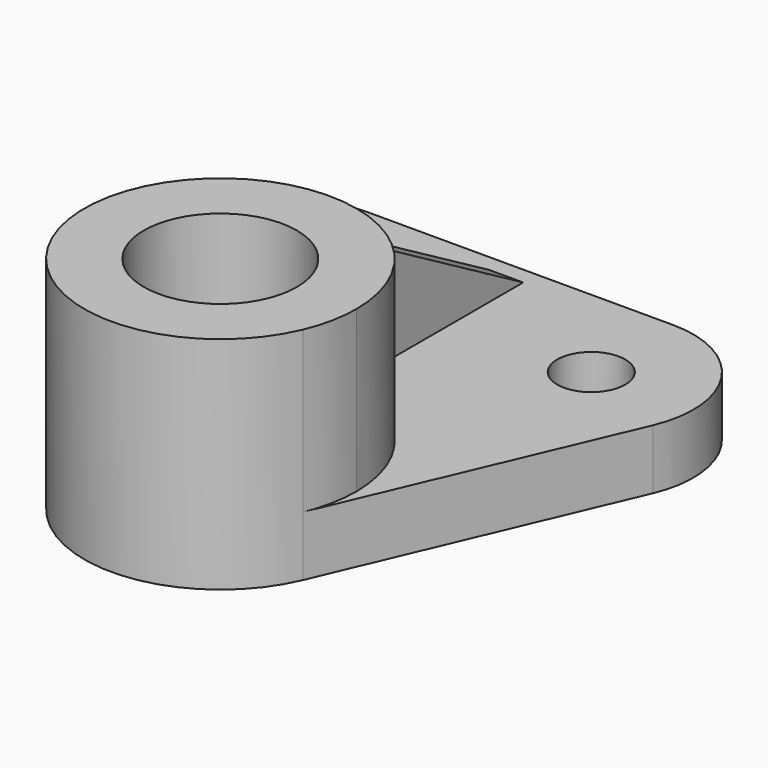
from build123d import *

# Parameters (mm, degrees)
F0_R     = 14.2875
F1_DEPTH = 41.148
F0_R_2   = 6.35
F2_DEPTH = 11.176
F4_DEPTH = 3.175


# Not quite as in the source:
# - a feature of the source that left no trace in its solid (it failed there, or was rolled back) is left out


with BuildPart() as f1:
    # F0 (on Top) → F1 (new body)
    with BuildSketch(Plane.XY):
        with BuildLine():
            ThreePointArc((23.3629201096, -9.9666425617), (24.8855195926, -5.0863458994), (25.4, 0))
            ThreePointArc((25.4, 0), (-5.0863458994, 24.8855195926), (-23.3629201096, -9.9666425617))
            ThreePointArc((-23.3629201096, -9.9666425617), (0, -25.4), (23.3629201096, -9.9666425617))
        make_face()
        Circle(F0_R, mode=Mode.SUBTRACT)
    extrude(amount=F1_DEPTH)

    # F0 (on Top) → F2 (join)
    with BuildSketch(Plane.XY):
        with BuildLine():
            ThreePointArc((-23.3629201096, -9.9666425617), (-5.0863458994, 24.8855195926), (25.4, 0))
            ThreePointArc((25.4, 0), (24.8855195926, -5.0863458994), (23.3629201096, -9.9666425617))
            Line((23.3629201096, -9.9666425617), (46.0971900822, 43.3250180788))
            ThreePointArc((46.0971900822, 43.3250180788), (44.4699820006, 61.3000974853), (28.575, 69.85))
            Line((28.575, 69.85), (-28.575, 69.85))
            ThreePointArc((-28.575, 69.85), (-44.4699820006, 61.3000974853), (-46.0971900822, 43.3250180788))
            Line((-46.0971900822, 43.3250180788), (-23.3629201096, -9.9666425617))
        make_face()
        with Locations((-28.575, 50.8)):
            Circle(F0_R_2, mode=Mode.SUBTRACT)
        with Locations((28.575, 50.8)):
            Circle(F0_R_2, mode=Mode.SUBTRACT)
    extrude(amount=F2_DEPTH)

    # F3 (on Right) → F4 (join, symmetric)
    with BuildSketch(Plane.YZ):
        Polygon((66.675, 11.176), (25.4, 35.0061323608), (25.4, 11.176), align=None)
        Polygon((25.4, 11.176), (25.4, 35.0061323608), (22.225, 36.8392194655), (22.225, 11.176), align=None)
    extrude(amount=F4_DEPTH, both=True)


solid = f1.part
